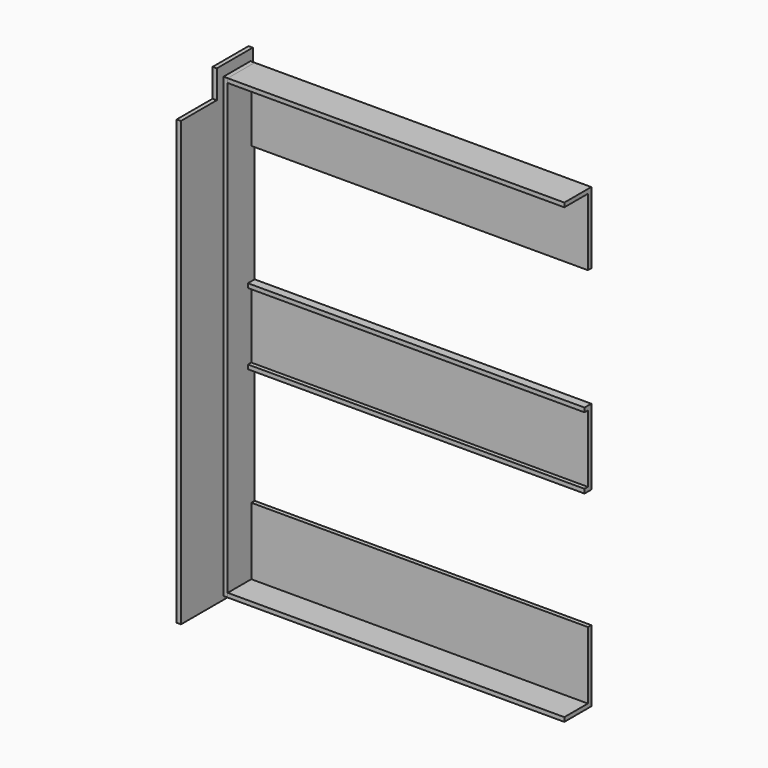
from build123d import *

# Parameters (mm, degrees)
F1_DEPTH = 19.05
F3_W     = 152.4
F3_H     = 19.05
F3_H_2   = 2032
F4_DEPTH = 19.05
F5_W     = 19.05
F5_H     = 304.8
F6_DEPTH = 1524


# Not quite as in the source:
# - a length typed as a fraction of an inch, garbled in the dataset ("3 / 203.2 mm" for 3/8 in), is restored
# - the program builds the solid bodies; features that only make, move or delete a surface that nothing else refers to are left out


with BuildPart() as f1:
    # F0 (on Right) → F1 (new body)
    with BuildSketch(Plane.YZ):
        Polygon((-406.4, 0), (0, 0), (0, 2133.6), (-203.2, 2133.6), (-203.2, 2006.6), (-406.4, 2006.6), align=None)
    extrude(amount=F1_DEPTH)


with BuildPart() as f4:
    # F3 (on offset) → F4 (new body)
    with BuildSketch(Plane.YZ.offset(23.8125)):
        with Locations((-95.25, 28.575)):
            Rectangle(F3_W, F3_H)
        with Locations((-95.25, 1054.1)):
            Rectangle(F3_W, F3_H_2)
        with Locations((-95.25, 2079.625)):
            Rectangle(F3_W, F3_H)
    extrude(amount=F4_DEPTH)


with BuildPart() as f6:
    # F5 (on face) → F6 (new body)
    with BuildSketch(Plane.YZ.offset(42.8625)):
        with Locations((-28.575, 1917.7)):
            Rectangle(F5_W, F5_H)
        Polygon((-38.1, 2070.1), (-19.05, 2070.1), (-19.05, 2089.15), (-171.45, 2089.15), (-171.45, 2070.1), align=None)
    extrude(amount=F6_DEPTH)


with BuildPart() as f6b:
    # F5 (on face) → F6, piece 2 (new body)
    with BuildSketch(Plane.YZ.offset(42.8625)):
        Polygon((-19.05, 19.05), (-19.05, 38.1), (-38.1, 38.1), (-171.45, 38.1), (-171.45, 19.05), align=None)
        with Locations((-28.575, 190.5)):
            Rectangle(F5_W, F5_H)
    extrude(amount=F6_DEPTH)


with BuildPart() as f6c:
    # F5 (on face) → F6, piece 3 (new body)
    with BuildSketch(Plane.YZ.offset(42.8625)):
        with Locations((-28.575, 1054.1)):
            Rectangle(F5_W, F5_H)
        Polygon((-38.1, 1206.5), (-19.05, 1206.5), (-19.05, 1225.55), (-57.15, 1225.55), (-57.15, 1206.5), align=None)
        Polygon((-19.05, 882.65), (-19.05, 901.7), (-38.1, 901.7), (-57.15, 901.7), (-57.15, 882.65), align=None)
    extrude(amount=F6_DEPTH)


solid = Compound([f1.part, f4.part, f6.part, f6b.part, f6c.part])
